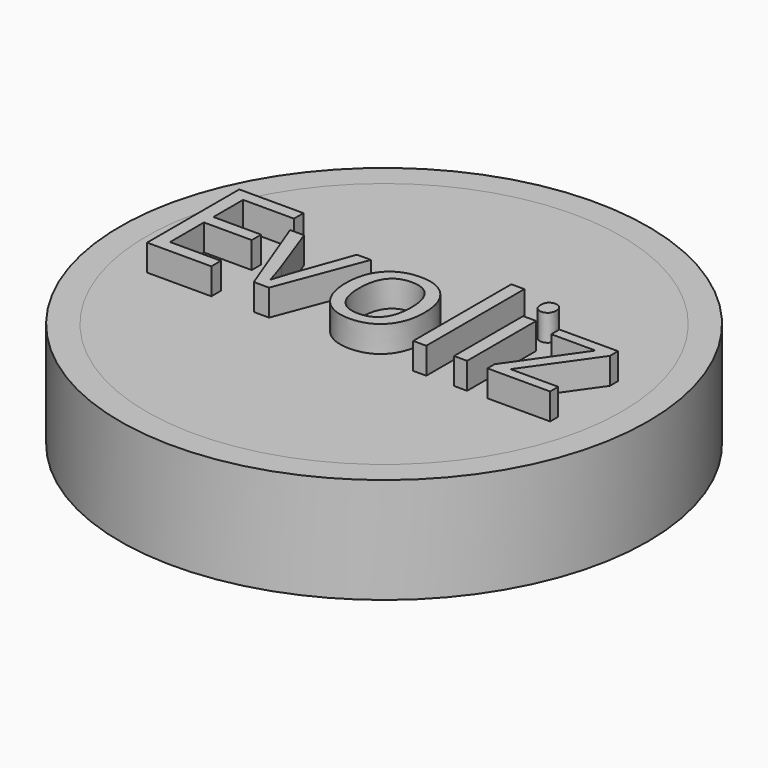
from build123d import *

# Parameters (mm, degrees)
F0_R         = 13.5
F1_DEPTH     = 3
F0_R_2       = 15
F2_DEPTH     = 6
F3_TEXT_SIZE = 9.1712323612
F4_DEPTH     = 1.5


# Not quite as in the source:
# - Text() gives the source's letters only with a copy of the font that has no kerning and outlines rounded to 1/6400 em; it was checked with that copy


with BuildPart() as f1:
    # F0 (on Top) → F1 (new body)
    with BuildSketch(Plane.XY):
        Circle(F0_R)
    extrude(amount=-F1_DEPTH)

    # F3 (on face) → F4 (join)
    with BuildSketch(Plane.XY):
        with Locations((-12.198455543, -2.7120269369)):
            Text('Evoliz', F3_TEXT_SIZE, font='Open Sans', text_align=(TextAlign.LEFT, TextAlign.BOTTOM))
    extrude(amount=F4_DEPTH)


with BuildPart() as f2:
    # F0 (on Top) → F2 (new body)
    with BuildSketch(Plane.XY):
        Circle(F0_R_2)
        Circle(F0_R, mode=Mode.SUBTRACT)
    extrude(amount=-F2_DEPTH)


solid = Compound([f1.part, f2.part])
